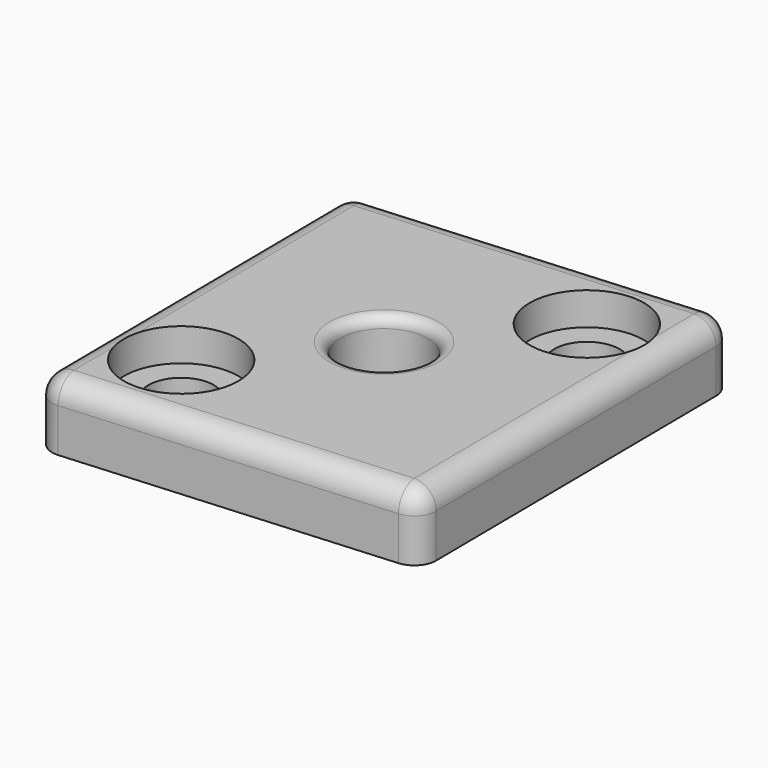
from build123d import *

# Parameters (mm, degrees)
F0_R         = 1.5
F0_R_2       = 2
F1_DEPTH     = 3
F2_R         = 2.625
F2_R_2       = 1.5
F3_DEPTH     = 1.5
F4_T1_DEPTH  = 4.3472443006
F4_T3_DEPTH  = 16.2344954865
F4_T5_DEPTH  = 14.8006020278
F4_T7_DEPTH  = 4.6626968477
F4_T9_DEPTH  = 16.2344954865
F4_T11_DEPTH = 14.8006020278
F4_T16_DEPTH = 1
F4_T22_DEPTH = 1
F4_T28_DEPTH = 1
F4_T34_DEPTH = 1
F5_R         = 0.5


# Not quite as in the source:
# - a fillet or chamfer that OpenCascade refuses, or shapes differently, is made with other operations: its cross-section is extruded or revolved along the edge and cut away or added


with BuildPart() as f1:
    # F0 (on Top) → F1 (new body)
    with BuildSketch(Plane.XY):
        Polygon((8.4645454874, -8.5124193832), (8.2962074114, 9.7252756798), (-8.4645454874, 8.5124193832), (-8.2962074114, -9.7252756798), align=None)
        with Locations((-4.8033426305, -5.6307453454)):
            Circle(F0_R, mode=Mode.SUBTRACT)
        Polygon((4.02705255, 0.3354530665), (2.3040371523, -3.3198032774), (-1.7230153977, -3.6552563439), (-4.02705255, -0.3354530665), (-2.3040371523, 3.3198032774), (1.7230153977, 3.6552563439), align=None, mode=Mode.SUBTRACT)
        with Locations((4.8033426305, 5.6307453454)):
            Circle(F0_R, mode=Mode.SUBTRACT)
        Polygon((-1.7230153977, -3.6552563439), (2.3040371523, -3.3198032774), (4.02705255, 0.3354530665), (1.7230153977, 3.6552563439), (-2.3040371523, 3.3198032774), (-4.02705255, -0.3354530665), align=None)
        Circle(F0_R_2, mode=Mode.SUBTRACT)
    extrude(amount=F1_DEPTH)

    # F2 (on face) → F3 (cut)
    with BuildSketch(Plane.XY.offset(3)):
        with Locations((-4.8033426305, -5.6307453454)):
            Circle(F2_R)
        with Locations((-4.8033426305, -5.6307453454)):
            Circle(F2_R_2, mode=Mode.SUBTRACT)
        with Locations((4.8033426305, 5.6307453454)):
            Circle(F2_R)
        with Locations((4.8033426305, 5.6307453454)):
            Circle(F2_R_2, mode=Mode.SUBTRACT)
    extrude(amount=-F3_DEPTH, mode=Mode.SUBTRACT)

    # F4: fillet of radius 1 on 8 edges, made by hand

    # F4_s2 → F4_t1 (cut)
    with BuildSketch(Plane.XY.offset(-2.3472443006)):
        with BuildLine():
            ThreePointArc((-7.5280963703, 8.5801835352), (-8.1912373991, 8.2605167863), (-8.4558796169, 7.573561656))
            Line((-8.4558796169, 7.573561656), (-8.4645454874, 8.5124193832))
            Line((-8.4645454874, 8.5124193832), (-7.5280963703, 8.5801835352))
        make_face()
        with BuildLine():
            ThreePointArc((8.4558796169, -7.573561656), (8.1912373991, -8.2605167863), (7.5280963703, -8.5801835352))
            Line((7.5280963703, -8.5801835352), (8.4645454874, -8.5124193832))
            Line((8.4645454874, -8.5124193832), (8.4558796169, -7.573561656))
        make_face()
    extrude(amount=F4_T1_DEPTH, mode=Mode.SUBTRACT)

    # F4_s4 → F4_t3 (cut)
    with BuildSketch(Plane(origin=(-0.0706200975, 7.6509595097, 0), x_dir=(0, 0, 1), z_dir=(0.0092298344, -0.9999574042, 0))):
        with BuildLine():
            ThreePointArc((3, 7.3856167117), (2.7071067812, 8.0927234929), (2, 8.3856167117))
            Line((2, 8.3856167117), (3, 8.3856167117))
            Line((3, 8.3856167117), (3, 7.3856167117))
        make_face()
    extrude(amount=F4_T3_DEPTH, mode=Mode.SUBTRACT)

    # F4_s6 → F4_t5 (cut)
    with BuildSketch(Plane(origin=(7.8907735218, 0.570999072, 0), x_dir=(0, 0, 1), z_dir=(-0.9973920448, -0.0721741576, 0))):
        with BuildLine():
            ThreePointArc((2, 9.1011408148), (2.7071067812, 8.808247596), (3, 8.1011408148))
            Line((3, 8.1011408148), (3, 9.1011408148))
            Line((3, 9.1011408148), (2, 9.1011408148))
        make_face()
    extrude(amount=F4_T5_DEPTH, mode=Mode.SUBTRACT)

    # F4_s8 → F4_t7 (cut)
    with BuildSketch(Plane.XY.offset(-2.6626968477)):
        with BuildLine():
            ThreePointArc((8.3060379118, 8.6602423087), (7.9838058035, 9.3863276607), (7.23390635, 9.648404519))
            Line((7.23390635, 9.648404519), (8.2962074114, 9.7252756798))
            Line((8.2962074114, 9.7252756798), (8.3060379118, 8.6602423087))
        make_face()
        with BuildLine():
            ThreePointArc((-7.23390635, -9.648404519), (-7.9838058035, -9.3863276607), (-8.3060379118, -8.6602423087))
            Line((-8.3060379118, -8.6602423087), (-8.2962074114, -9.7252756798))
            Line((-8.2962074114, -9.7252756798), (-7.23390635, -9.648404519))
        make_face()
    extrude(amount=F4_T7_DEPTH, mode=Mode.SUBTRACT)

    # F4_s10 → F4_t9 (cut)
    with BuildSketch(Plane(origin=(0.0706200975, -7.6509595097, 0), x_dir=(0, 0, 1), z_dir=(-0.0092298344, 0.9999574042, 0))):
        with BuildLine():
            ThreePointArc((2, 8.3856167117), (2.7071067812, 8.0927234929), (3, 7.3856167117))
            Line((3, 7.3856167117), (3, 8.3856167117))
            Line((3, 8.3856167117), (2, 8.3856167117))
        make_face()
    extrude(amount=F4_T9_DEPTH, mode=Mode.SUBTRACT)

    # F4_s12 → F4_t11 (cut)
    with BuildSketch(Plane(origin=(-7.8907735218, -0.570999072, 0), x_dir=(0, 0, 1), z_dir=(0.9973920448, 0.0721741576, 0))):
        with BuildLine():
            ThreePointArc((2, 9.1011408148), (2.7071067812, 8.808247596), (3, 8.1011408148))
            Line((3, 8.1011408148), (3, 9.1011408148))
            Line((3, 9.1011408148), (2, 9.1011408148))
        make_face()
    extrude(amount=F4_T11_DEPTH, mode=Mode.SUBTRACT)


with BuildPart() as f4_tool14:
    # F4_s15 → F4_t16 (new body)
    with BuildSketch(Plane.XY.offset(2)):
        Polygon((-7.4559222127, 7.5827914904), (-8.4558796169, 7.573561656), (-8.4645454874, 8.5124193832), (-7.5280963703, 8.5801835352), align=None)
    extrude(amount=F4_T16_DEPTH)

    # F4_s17 → F4_t18 (revolve, cut)
    with BuildSketch(Plane(origin=(-7.4559222127, 7.5827914904, 2), x_dir=(0.7353151864, -0.6777252959, 0), z_dir=(-0.6777252959, -0.7353151864, 0))):
        with BuildLine():
            ThreePointArc((0, -1), (1, 0), (0, 1))
            Line((0, 1), (0, -1))
        make_face()
    revolve(axis=Axis((-7.4559222127, 7.5827914904, 2), (0, 0, 1)), mode=Mode.SUBTRACT)


with BuildPart() as f1_1:
    add(f1.part)

    # F4_t13: cut F4_tool14
    add(f4_tool14.part, mode=Mode.SUBTRACT)


with BuildPart() as f4_tool20:
    # F4_s21 → F4_t22 (new body)
    with BuildSketch(Plane.XY.offset(2)):
        Polygon((-7.3060805076, -8.6510124742), (-8.3060379118, -8.6602423087), (-8.2962074114, -9.7252756798), (-7.23390635, -9.648404519), align=None)
    extrude(amount=F4_T22_DEPTH)

    # F4_s23 → F4_t24 (revolve, cut)
    with BuildSketch(Plane(origin=(-7.3060805076, -8.6510124742, 2), x_dir=(0.6777252959, 0.7353151864, 0), z_dir=(0.7353151864, -0.6777252959, 0))):
        with BuildLine():
            ThreePointArc((0, -1), (1, 0), (0, 1))
            Line((0, 1), (0, -1))
        make_face()
    revolve(axis=Axis((-7.3060805076, -8.6510124742, 2), (0, 0, 1)), mode=Mode.SUBTRACT)


with BuildPart() as f1_2:
    add(f1_1.part)

    # F4_t19: cut F4_tool20
    add(f4_tool20.part, mode=Mode.SUBTRACT)


with BuildPart() as f4_tool26:
    # F4_s27 → F4_t28 (new body)
    with BuildSketch(Plane.XY.offset(2)):
        Polygon((7.3060805076, 8.6510124742), (8.3060379118, 8.6602423087), (8.2962074114, 9.7252756798), (7.23390635, 9.648404519), align=None)
    extrude(amount=F4_T28_DEPTH)

    # F4_s29 → F4_t30 (revolve, cut)
    with BuildSketch(Plane(origin=(7.3060805076, 8.6510124742, 2), x_dir=(-0.6777252959, -0.7353151864, 0), z_dir=(-0.7353151864, 0.6777252959, 0))):
        with BuildLine():
            ThreePointArc((0, -1), (1, 0), (0, 1))
            Line((0, 1), (0, -1))
        make_face()
    revolve(axis=Axis((7.3060805076, 8.6510124742, 2), (0, 0, 1)), mode=Mode.SUBTRACT)


with BuildPart() as f1_3:
    add(f1_2.part)

    # F4_t25: cut F4_tool26
    add(f4_tool26.part, mode=Mode.SUBTRACT)


with BuildPart() as f4_tool32:
    # F4_s33 → F4_t34 (new body)
    with BuildSketch(Plane.XY.offset(2)):
        Polygon((7.4559222127, -7.5827914904), (8.4558796169, -7.573561656), (8.4645454874, -8.5124193832), (7.5280963703, -8.5801835352), align=None)
    extrude(amount=F4_T34_DEPTH)

    # F4_s35 → F4_t36 (revolve, cut)
    with BuildSketch(Plane(origin=(7.4559222127, -7.5827914904, 2), x_dir=(-0.7353151864, 0.6777252959, 0), z_dir=(0.6777252959, 0.7353151864, 0))):
        with BuildLine():
            ThreePointArc((0, -1), (1, 0), (0, 1))
            Line((0, 1), (0, -1))
        make_face()
    revolve(axis=Axis((7.4559222127, -7.5827914904, 2), (0, 0, 1)), mode=Mode.SUBTRACT)


with BuildPart() as f1_4:
    add(f1_3.part)

    # F4_t31: cut F4_tool32
    add(f4_tool32.part, mode=Mode.SUBTRACT)

    # F5
    f5_edges = [f1_4.edges().sort_by_distance(p)[0] for p in [
        (-2, 0, 3),
    ]]
    fillet(f5_edges, radius=F5_R)


solid = f1_4.part
